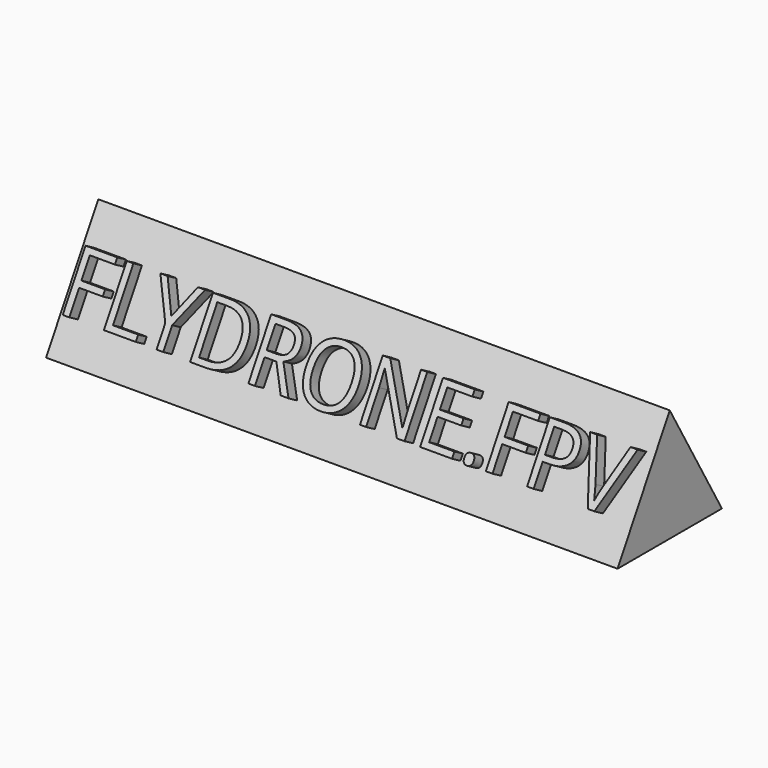
from build123d import *

# Parameters (mm, degrees)
F1_DEPTH     = 46
F2_TEXT_SIZE = 6.4296172544
F3_DEPTH     = 1


# Not quite as in the source:
# - Text() gives the source's letters only with a copy of the font that has no kerning and outlines rounded to 1/6400 em; it was checked with that copy


with BuildPart() as f1:
    # F0 (on Right) → F1 (new body)
    with BuildSketch(Plane.YZ):
        Polygon((0, 6.0621778265), (-5.25, -3.0310889132), (5.25, -3.0310889132), align=None)
    extrude(amount=F1_DEPTH)

    # F2 (on face) → F3 (join)
    with BuildSketch(Plane(origin=(0, -2.625, 1.5155444566), x_dir=(1, 0, 0), z_dir=(0, -0.8660254038, 0.5))):
        with Locations((0.2196892747, -2.2983909585)):
            Text('FLYDRONE.FPV', F2_TEXT_SIZE, font='Open Sans', text_align=(TextAlign.LEFT, TextAlign.BOTTOM))
    extrude(amount=F3_DEPTH)


solid = f1.part
